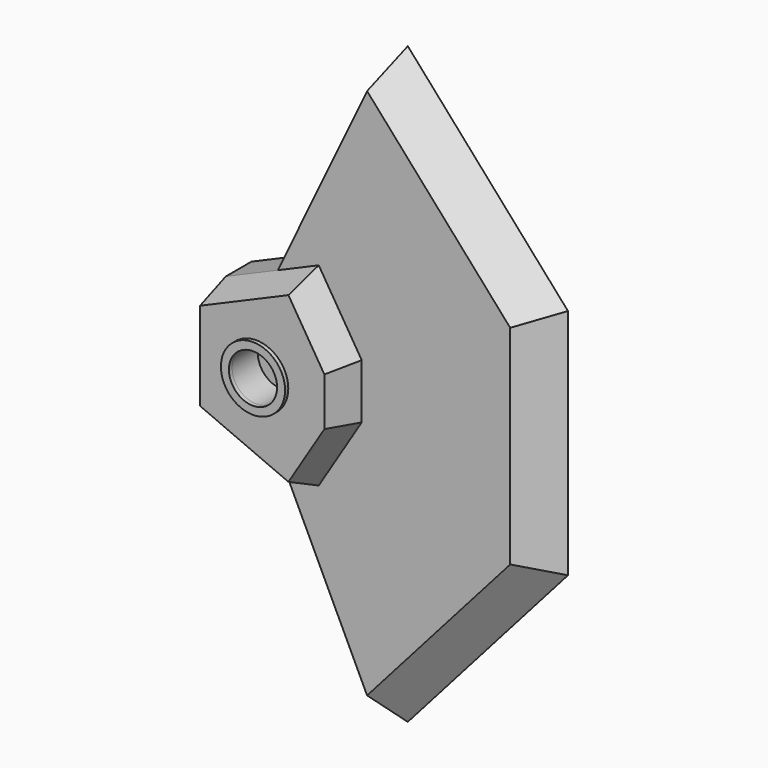
from build123d import *

# Parameters (mm, degrees)
F1_DEPTH      = 8
F1_TAPER      = -20
F2_W          = 14.830423519
F2_H          = 54.1627034545
F3_DEPTH      = 8.0010001
F4_R          = 6
F5_DEPTH      = 8.0010001
F5_DEPTH_BACK = 77
F4_R_2        = 8
F6_DEPTH      = 1
F9_DEPTH      = 8
F10_SIZE      = 7.99999


# Not quite as in the source:
# - a fillet or chamfer is up to 0.001 mm smaller than in the source, because OpenCascade refuses the exact size
# - an extrude ends at something that could not be found from the text; its depth is read off the source's solid


with BuildPart() as f1:
    # F0 (on Front) → F1 (new body)
    with BuildSketch(Plane.XZ):
        Polygon((0, 11), (0, 0), (0, -11), (22.0397368405, -20.5), (31, -6), (31, 0), (31, 6), (22.0397368405, 20.5), align=None)
    extrude(amount=-F1_DEPTH, taper=F1_TAPER)

    # F2 (on Front) → F3 (cut, through all)
    with BuildSketch(Plane.XZ):
        with Locations((-7.4152117595, -1.4976877719)):
            Rectangle(F2_W, F2_H)
    extrude(amount=-F3_DEPTH, mode=Mode.SUBTRACT)

    # F4 (on Front) → F5 (cut, two sides)
    with BuildSketch(Plane.XZ) as f5_sk:
        with Locations((14, 0)):
            Circle(F4_R)
    extrude(amount=-F5_DEPTH, mode=Mode.SUBTRACT)
    extrude(f5_sk.sketch, amount=F5_DEPTH_BACK, mode=Mode.SUBTRACT)

    # F4 (on Front) → F6 (join)
    with BuildSketch(Plane.XZ):
        with Locations((14, 0)):
            Circle(F4_R_2)
        with Locations((14, 0)):
            Circle(F4_R, mode=Mode.SUBTRACT)
    extrude(amount=F6_DEPTH)

    # F8 (on face) → F9 (join)
    with BuildSketch(Plane(origin=(0, 8, 0), x_dir=(-1, 0, 0), z_dir=(0, 1, 0))):
        Polygon((-39, -74.1707404442), (-13, -19.7742556265), (0, -14.1707404442), (0, 14.1707404442), (-13, 19.7742556265), (-39, 74.1707404442), (-78.9322146674, 29), (-78.9322146674, -29), align=None)
    extrude(amount=F9_DEPTH)

    # F10 (size 8 in the source; OpenCascade refuses exactly that, so slightly less here)
    f10_edges = [f1.edges().sort_by_distance(p)[0] for p in [
        (58.966107, 8, 51.58537),
        (78.932215, 8, 0),
        (58.966107, 8, -51.58537),
    ]]
    chamfer(f10_edges, length=F10_SIZE)


solid = f1.part
